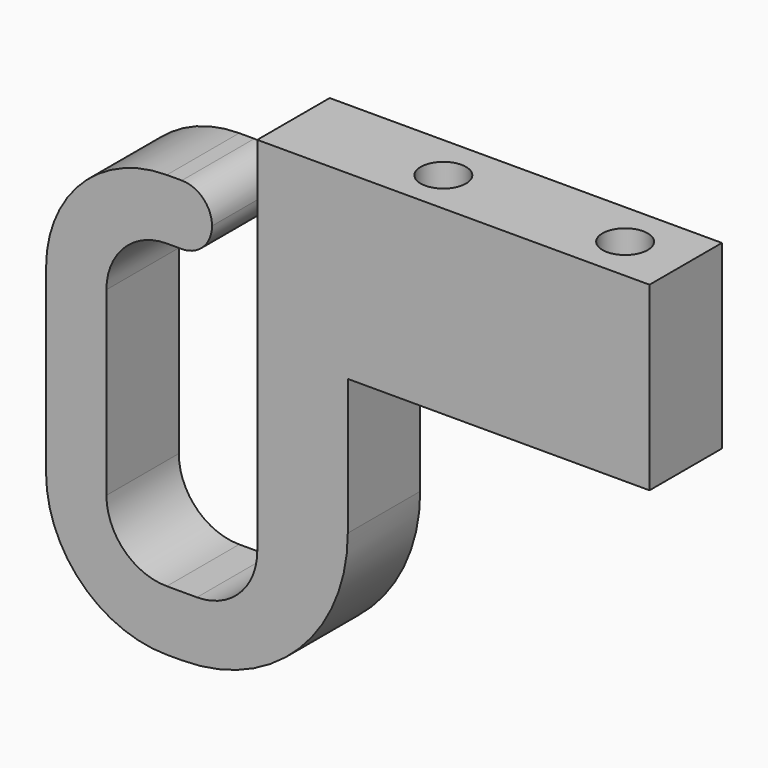
from build123d import *

# Parameters (mm, degrees)
F1_DEPTH       = 6
F2_R           = 4
F3_R           = 8
F4_R           = 11
F5_R           = 1.99999
F7_D           = 3
F7_CSINK_D     = 5
F7_CSINK_ANGLE = 90


# Not quite as in the source:
# - a fillet or chamfer is up to 0.001 mm smaller than in the source, because OpenCascade refuses the exact size


with BuildPart() as f1:
    # F0 (on Front) → F1 (new body)
    with BuildSketch(Plane.XZ):
        Polygon((0, 0), (0, 20), (7, 20), (7, 24), (-4, 24), (-4, -4), (16, -4), (16, 16), (36, 16), (36, 28), (10, 28), (10, 0), align=None)
    extrude(amount=F1_DEPTH)

    # F2
    f2_edges = [f1.edges().sort_by_distance(p)[0] for p in [
        (10, -3, 0),
        (0, -3, 0),
        (0, -3, 20),
    ]]
    fillet(f2_edges, radius=F2_R)

    # F3
    f3_edges = [f1.edges().sort_by_distance(p)[0] for p in [
        (-4, -3, 24),
        (-4, -3, -4),
    ]]
    fillet(f3_edges, radius=F3_R)

    # F4
    f4_edges = [f1.edges().sort_by_distance(p)[0] for p in [
        (16, -3, -4),
    ]]
    fillet(f4_edges, radius=F4_R)

    # F5 (radius 2 in the source; OpenCascade refuses exactly that, so slightly less here)
    f5_edges = [f1.edges().sort_by_distance(p)[0] for p in [
        (7, -3, 24),
        (7, -3, 20),
    ]]
    fillet(f5_edges, radius=F5_R)

    # F7 (through all)
    with Locations(Plane(origin=(0, 0, 16), x_dir=(1, 0, 0), z_dir=(0, 0, -1))):
        with Locations((20, 3.0815127769), (31.9998442765, 3.0203789876)):
            CounterSinkHole(F7_D / 2, F7_CSINK_D / 2, counter_sink_angle=F7_CSINK_ANGLE)


solid = f1.part
